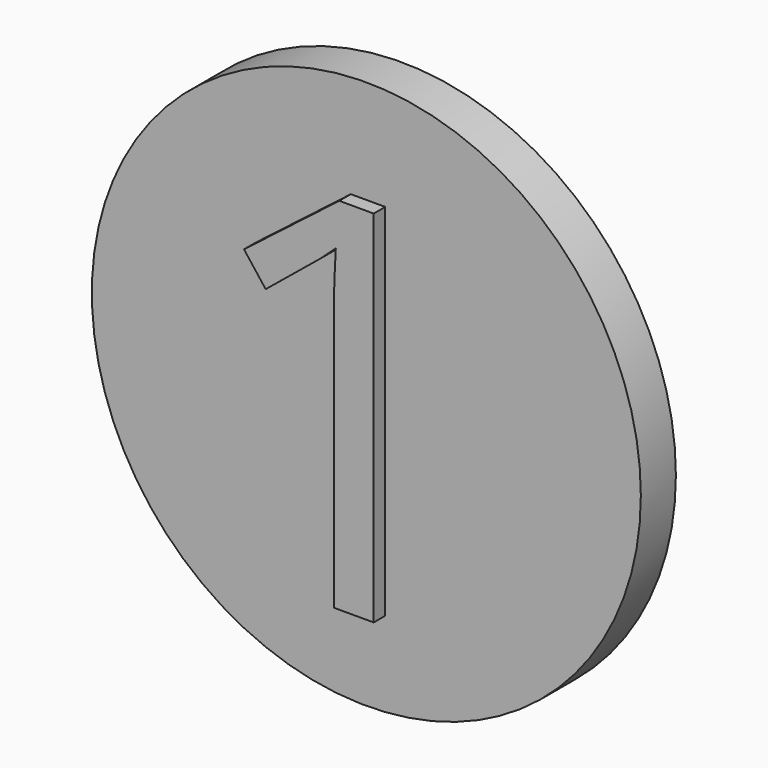
from build123d import *

# Parameters (mm, degrees)
F0_R         = 9.525
F1_DEPTH     = 1.52
F2_TEXT_SIZE = 17.4963523427
F3_DEPTH     = 0.5


# Not quite as in the source:
# - Text() gives the source's letters only with a copy of the font that has no kerning and outlines rounded to 1/6400 em; it was checked with that copy


with BuildPart() as f1:
    # F0 (on Front) → F1 (new body)
    with BuildSketch(Plane.XZ):
        Circle(F0_R)
    extrude(amount=F1_DEPTH)

    # F2 (on face) → F3 (join)
    with BuildSketch(Plane.XZ.offset(1.52)):
        with Locations((-5.4518915713, -6.5594898952)):
            Text('1', F2_TEXT_SIZE, font='Open Sans', text_align=(TextAlign.LEFT, TextAlign.BOTTOM))
    extrude(amount=F3_DEPTH)


solid = f1.part
